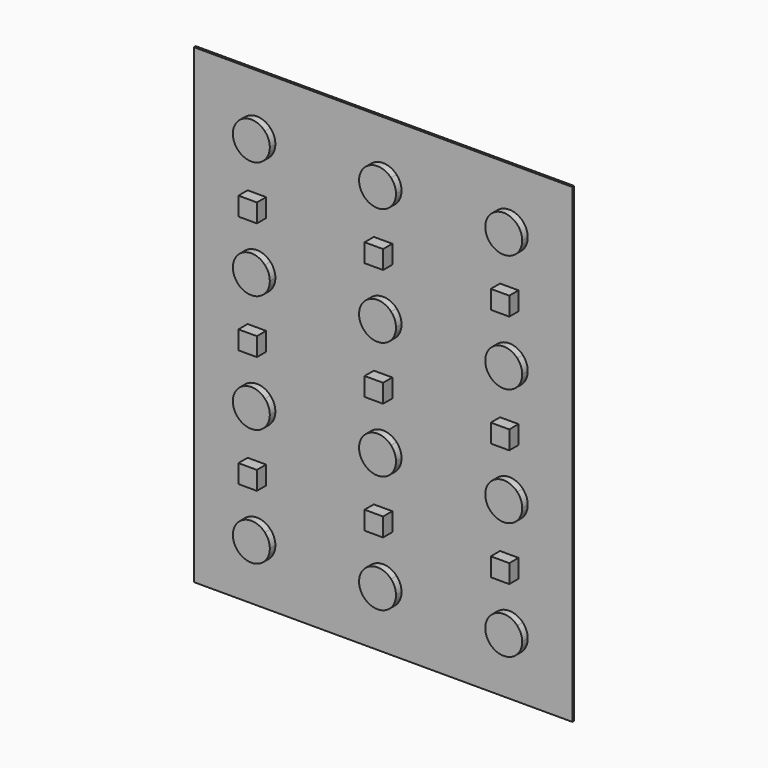
from build123d import *

# Parameters (mm, degrees)
F1_DEPTH = 3.175
F2_DEPTH = 12.7
F0_W     = 25.4
F0_H     = 12.7
F3_DEPTH = 19.05


# Not quite as in the source:
# - ends of sketch curves that miss each other by under 0.0002 mm in the source are joined


with BuildPart() as f1:
    # F0 (on Front) → F1 (new body)
    with BuildSketch(Plane.XZ):
        Polygon((-86.7833418, 323.85), (-260.35, 323.85), (-260.35, 161.925), (-186.2666709, 161.925), (-186.2666709, 174.625), (-160.8666709, 174.625), (-160.8666709, 161.925), (-86.7833418, 161.925), align=None)
        with BuildLine():
            ThreePointArc((-148.1666709, 242.8875), (-149.9350898056, 233.5757668112), (-154.9941020007, 225.5606513402))
            ThreePointArc((-154.9941020007, 225.5606513402), (-173.5666709, 217.4875), (-192.1392397993, 225.5606513402))
            ThreePointArc((-192.1392397993, 225.5606513402), (-198.9666709, 242.8875), (-192.1392397993, 260.2143486598))
            ThreePointArc((-192.1392397993, 260.2143486598), (-173.5666709, 268.2875), (-154.9941020007, 260.2143486598))
            ThreePointArc((-154.9941020007, 260.2143486598), (-149.9350898056, 252.1992331888), (-148.1666709, 242.8875))
        make_face(mode=Mode.SUBTRACT)
        Polygon((-186.2666709, 161.925), (-260.35, 161.925), (-260.35, 0), (-186.2666709, 0), (-186.2666709, 12.7), (-160.8666709, 12.7), (-160.8666709, 0), (-86.7833418, 0), (-86.7833418, 161.925), (-160.8666709, 161.925), (-160.8666709, 149.225), (-186.2666709, 149.225), align=None)
        with BuildLine():
            ThreePointArc((-154.9941020007, 63.6356513402), (-173.5666709, 55.5625), (-192.1392397993, 63.6356513402))
            ThreePointArc((-192.1392397993, 63.6356513402), (-198.9666709, 80.9625), (-192.1392397993, 98.2893486598))
            ThreePointArc((-192.1392397993, 98.2893486598), (-173.5666709, 106.3625), (-154.9941020007, 98.2893486598))
            ThreePointArc((-154.9941020007, 98.2893486598), (-149.9350898056, 90.2742331888), (-148.1666709, 80.9625))
            ThreePointArc((-148.1666709, 80.9625), (-149.9350898056, 71.6507668112), (-154.9941020007, 63.6356513402))
        make_face(mode=Mode.SUBTRACT)
        Polygon((-12.7, 161.925), (-86.7833418, 161.925), (-86.7833418, 0), (-12.7, 0), (-12.7, 12.7), (12.7, 12.7), (12.7, 0), (86.78332402, 0), (86.78332402, 161.925), (12.7, 161.925), (12.7, 149.225), (-12.7, 149.225), align=None)
        with BuildLine():
            ThreePointArc((18.5725583517, 63.6356536473), (-1.11224e-05, 55.5625), (-18.5725815993, 63.6356513402))
            ThreePointArc((-18.5725815993, 63.6356513402), (-25.4000127, 80.9625010214), (-18.5725802058, 98.2893501535))
            ThreePointArc((-18.5725802058, 98.2893501535), (-1.16786e-05, 106.3625), (18.5725561993, 98.2893486598))
            ThreePointArc((18.5725561993, 98.2893486598), (23.6315683944, 90.2742331888), (25.3999873, 80.9625))
            ThreePointArc((25.3999873, 80.9625), (23.6315689728, 71.650768279), (18.5725583517, 63.6356536473))
        make_face(mode=Mode.SUBTRACT)
        Polygon((86.78332402, 323.85), (-86.7833418, 323.85), (-86.7833418, 161.925), (-12.7, 161.925), (-12.7, 174.625), (12.7, 174.625), (12.7, 161.925), (86.78332402, 161.925), align=None)
        with BuildLine():
            ThreePointArc((25.399989205, 242.8874982228), (23.6315702994, 233.575765034), (18.5725581043, 225.560649563))
            ThreePointArc((18.5725581043, 225.560649563), (-1.10731e-05, 217.4874982228), (-18.5725800737, 225.5606499697))
            ThreePointArc((-18.5725800737, 225.5606499697), (-17.3268590481, 261.4600675015), (18.5725584837, 260.2143464759))
            ThreePointArc((18.5725584837, 260.2143464759), (23.6315704014, 252.1992311528), (25.399989205, 242.8874982228))
        make_face(mode=Mode.SUBTRACT)
        Polygon((260.35, 323.85), (86.78332402, 323.85), (86.78332402, 161.925), (160.86666201, 161.925), (160.86666201, 174.625), (186.26666201, 174.625), (186.26666201, 161.925), (260.35, 161.925), align=None)
        with BuildLine():
            ThreePointArc((198.96666201, 242.8875), (182.8783931272, 219.2559180893), (154.994090073, 225.5606545963))
            ThreePointArc((154.994090073, 225.5606545963), (148.16666201, 242.8875015776), (154.9940922253, 260.2143477108))
            ThreePointArc((154.9940922253, 260.2143477108), (173.5666609886, 268.2875), (192.1392304011, 260.2143492045))
            ThreePointArc((192.1392304011, 260.2143492045), (197.1982429678, 252.1992335353), (198.96666201, 242.8875))
        make_face(mode=Mode.SUBTRACT)
        Polygon((160.86666201, 0), (86.78332402, 0), (86.78332402, -161.925), (160.86666201, -161.925), (160.86666201, -149.225), (186.26666201, -149.225), (186.26666201, -161.925), (260.35, -161.925), (260.35, 0), (186.26666201, 0), (186.26666201, -12.7), (160.86666201, -12.7), align=None)
        with BuildLine():
            ThreePointArc((192.1392317947, -98.2893477108), (173.56666201, -106.3625), (154.9940922253, -98.2893477108))
            ThreePointArc((154.9940922253, -98.2893477108), (148.16666201, -80.9625), (154.9940922253, -63.6356522892))
            ThreePointArc((154.9940922253, -63.6356522892), (173.56666201, -55.5625), (192.1392317947, -63.6356522892))
            ThreePointArc((192.1392317947, -63.6356522892), (197.1982433423, -71.650767415), (198.96666201, -80.9625))
            ThreePointArc((198.96666201, -80.9625), (197.1982433423, -90.274232585), (192.1392317947, -98.2893477108))
        make_face(mode=Mode.SUBTRACT)
        Polygon((160.86666201, 161.925), (86.78332402, 161.925), (86.78332402, 0), (160.86666201, 0), (160.86666201, 12.7), (186.26666201, 12.7), (186.26666201, 0), (260.35, 0), (260.35, 161.925), (186.26666201, 161.925), (186.26666201, 149.225), (160.86666201, 149.225), align=None)
        with BuildLine():
            ThreePointArc((192.1392321741, 63.6356491414), (173.5666609886, 55.5624964455), (154.9940904524, 63.6356506351))
            ThreePointArc((154.9940904524, 63.6356506351), (148.16666201, 80.962497467), (154.9940918459, 98.2893437497))
            ThreePointArc((154.9940918459, 98.2893437497), (173.5666604324, 106.3624964455), (192.1392300217, 98.2893460568))
            ThreePointArc((192.1392300217, 98.2893460568), (197.1982428659, 90.2742302396), (198.96666201, 80.9624964455))
            ThreePointArc((198.96666201, 80.9624964455), (197.1982434443, 71.6507641193), (192.1392321741, 63.6356491414))
        make_face(mode=Mode.SUBTRACT)
        Polygon((-12.7, 0), (-86.7833418, 0), (-86.7833418, -161.925), (-12.7, -161.925), (-12.7, -149.225), (12.7, -149.225), (12.7, -161.925), (86.78332402, -161.925), (86.78332402, 0), (12.7, 0), (12.7, -12.7), (-12.7, -12.7), align=None)
        with BuildLine():
            ThreePointArc((18.5725603887, -98.2893482531), (-8.89e-06, -106.3625), (-18.5725781687, -98.2893482531))
            ThreePointArc((-18.5725781687, -98.2893482531), (-25.40000889, -80.9625), (-18.5725781687, -63.6356517469))
            ThreePointArc((-18.5725781687, -63.6356517469), (-8.89e-06, -55.5625), (18.5725603887, -63.6356517469))
            ThreePointArc((18.5725603887, -63.6356517469), (23.6315723064, -71.65076707), (25.39999111, -80.9625))
            ThreePointArc((25.39999111, -80.9625), (23.6315723064, -90.27423293), (18.5725603887, -98.2893482531))
        make_face(mode=Mode.SUBTRACT)
        Polygon((-186.2666709, 0), (-260.35, 0), (-260.35, -161.925), (-186.2666709, -161.925), (-186.2666709, -149.225), (-160.8666709, -149.225), (-160.8666709, -161.925), (-86.7833418, -161.925), (-86.7833418, 0), (-160.8666709, 0), (-160.8666709, -12.7), (-186.2666709, -12.7), align=None)
        with BuildLine():
            ThreePointArc((-154.9941020007, -98.2893486598), (-173.5666709, -106.3625), (-192.1392397993, -98.2893486598))
            ThreePointArc((-192.1392397993, -98.2893486598), (-198.9666709, -80.9625), (-192.1392397993, -63.6356513402))
            ThreePointArc((-192.1392397993, -63.6356513402), (-173.5666709, -55.5625), (-154.9941020007, -63.6356513402))
            ThreePointArc((-154.9941020007, -63.6356513402), (-149.9350898056, -71.6507668112), (-148.1666709, -80.9625))
            ThreePointArc((-148.1666709, -80.9625), (-149.9350898056, -90.2742331888), (-154.9941020007, -98.2893486598))
        make_face(mode=Mode.SUBTRACT)
        Polygon((-186.2666709, -161.925), (-260.35, -161.925), (-260.35, -323.85), (-86.7833418, -323.85), (-86.7833418, -161.925), (-160.8666709, -161.925), (-160.8666709, -174.625), (-186.2666709, -174.625), align=None)
        with BuildLine():
            ThreePointArc((-154.9941020007, -260.2143486598), (-173.5666709, -268.2875), (-192.1392397993, -260.2143486598))
            ThreePointArc((-192.1392397993, -260.2143486598), (-198.9666709, -242.8875), (-192.1392397993, -225.5606513402))
            ThreePointArc((-192.1392397993, -225.5606513402), (-173.5666709, -217.4875), (-154.9941020007, -225.5606513402))
            ThreePointArc((-154.9941020007, -225.5606513402), (-149.9350898056, -233.5757668112), (-148.1666709, -242.8875))
            ThreePointArc((-148.1666709, -242.8875), (-149.9350898056, -252.1992331888), (-154.9941020007, -260.2143486598))
        make_face(mode=Mode.SUBTRACT)
        Polygon((-12.7, -161.925), (-86.7833418, -161.925), (-86.7833418, -323.85), (86.78332402, -323.85), (86.78332402, -161.925), (12.7, -161.925), (12.7, -174.625), (-12.7, -174.625), align=None)
        with BuildLine():
            ThreePointArc((-18.5725781687, -260.2143482531), (-25.40000889, -242.8875), (-18.5725781687, -225.5606517469))
            ThreePointArc((-18.5725781687, -225.5606517469), (-8.89e-06, -217.4875), (18.5725603887, -225.5606517469))
            ThreePointArc((18.5725603887, -225.5606517469), (23.6315723064, -233.57576707), (25.39999111, -242.8875))
            ThreePointArc((25.39999111, -242.8875), (23.6315723064, -252.19923293), (18.5725603887, -260.2143482531))
            ThreePointArc((18.5725603887, -260.2143482531), (-8.89e-06, -268.2875), (-18.5725781687, -260.2143482531))
        make_face(mode=Mode.SUBTRACT)
        Polygon((160.86666201, -161.925), (86.78332402, -161.925), (86.78332402, -323.85), (260.35, -323.85), (260.35, -161.925), (186.26666201, -161.925), (186.26666201, -174.625), (160.86666201, -174.625), align=None)
        with BuildLine():
            ThreePointArc((154.9940922253, -225.5606522892), (173.56666201, -217.4875), (192.1392317947, -225.5606522892))
            ThreePointArc((192.1392317947, -225.5606522892), (197.1982433423, -233.575767415), (198.96666201, -242.8875))
            ThreePointArc((198.96666201, -242.8875), (197.1982433423, -252.199232585), (192.1392317947, -260.2143477108))
            ThreePointArc((192.1392317947, -260.2143477108), (173.56666201, -268.2875), (154.9940922253, -260.2143477108))
            ThreePointArc((154.9940922253, -260.2143477108), (148.16666201, -242.8875), (154.9940922253, -225.5606522892))
        make_face(mode=Mode.SUBTRACT)
    extrude(amount=F1_DEPTH)

    # F0 (on Front) → F2 (join)
    with BuildSketch(Plane.XZ):
        with BuildLine():
            Line((-192.1392397993, 260.2143486598), (-173.5666709, 242.8875))
            Line((-173.5666709, 242.8875), (-154.9941020007, 260.2143486598))
            ThreePointArc((-154.9941020007, 260.2143486598), (-173.5666709, 268.2875), (-192.1392397993, 260.2143486598))
        make_face()
        with BuildLine():
            Line((-192.1392397993, 225.5606513402), (-173.5666709, 242.8875))
            Line((-173.5666709, 242.8875), (-192.1392397993, 260.2143486598))
            ThreePointArc((-192.1392397993, 260.2143486598), (-198.9666709, 242.8875), (-192.1392397993, 225.5606513402))
        make_face()
        with BuildLine():
            ThreePointArc((-192.1392397993, 225.5606513402), (-173.5666709, 217.4875), (-154.9941020007, 225.5606513402))
            Line((-154.9941020007, 225.5606513402), (-173.5666709, 242.8875))
            Line((-173.5666709, 242.8875), (-192.1392397993, 225.5606513402))
        make_face()
        with BuildLine():
            Line((-173.5666709, 242.8875), (-154.9941020007, 225.5606513402))
            ThreePointArc((-154.9941020007, 225.5606513402), (-149.9350898056, 233.5757668112), (-148.1666709, 242.8875))
            ThreePointArc((-148.1666709, 242.8875), (-149.9350898056, 252.1992331888), (-154.9941020007, 260.2143486598))
            Line((-154.9941020007, 260.2143486598), (-173.5666709, 242.8875))
        make_face()
        with BuildLine():
            Line((-18.5725800737, 225.5606499697), (-1.0795e-05, 242.8874982228))
            Line((-1.0795e-05, 242.8874982228), (18.5725584837, 260.2143464759))
            ThreePointArc((18.5725584837, 260.2143464759), (-17.3268590481, 261.4600675015), (-18.5725800737, 225.5606499697))
        make_face()
        with BuildLine():
            Line((18.5725584837, 260.2143464759), (-1.0795e-05, 242.8874982228))
            Line((-1.0795e-05, 242.8874982228), (18.5725581043, 225.560649563))
            ThreePointArc((18.5725581043, 225.560649563), (23.6315702994, 233.575765034), (25.399989205, 242.8874982228))
            ThreePointArc((25.399989205, 242.8874982228), (23.6315704014, 252.1992311528), (18.5725584837, 260.2143464759))
        make_face()
        with BuildLine():
            Line((18.5725581043, 225.560649563), (-1.0795e-05, 242.8874982228))
            Line((-1.0795e-05, 242.8874982228), (-18.5725800737, 225.5606499697))
            ThreePointArc((-18.5725800737, 225.5606499697), (-1.10731e-05, 217.4874982228), (18.5725581043, 225.560649563))
        make_face()
        with BuildLine():
            Line((154.9940922253, 260.2143477108), (173.56666201, 242.8875))
            Line((173.56666201, 242.8875), (192.1392304011, 260.2143492045))
            ThreePointArc((192.1392304011, 260.2143492045), (173.5666609886, 268.2875), (154.9940922253, 260.2143477108))
        make_face()
        with BuildLine():
            ThreePointArc((154.9940922253, 260.2143477108), (148.16666201, 242.8875015776), (154.994090073, 225.5606545963))
            Line((154.994090073, 225.5606545963), (173.566660237, 242.8875019004))
            Line((173.566660237, 242.8875019004), (154.9940922253, 260.2143477108))
        make_face()
        with BuildLine():
            Line((173.566660237, 242.8875019004), (154.994090073, 225.5606545963))
            ThreePointArc((154.994090073, 225.5606545963), (182.8783931272, 219.2559180893), (198.96666201, 242.8875))
            ThreePointArc((198.96666201, 242.8875), (197.1982429678, 252.1992335353), (192.1392304011, 260.2143492045))
            Line((192.1392304011, 260.2143492045), (173.566660237, 242.8875019004))
        make_face()
        with BuildLine():
            Line((154.9940918459, 98.2893437497), (173.566660105, 80.9624982228))
            Line((173.566660105, 80.9624982228), (192.1392300217, 98.2893460568))
            ThreePointArc((192.1392300217, 98.2893460568), (173.5666604324, 106.3624964455), (154.9940918459, 98.2893437497))
        make_face()
        with BuildLine():
            ThreePointArc((154.9940918459, 98.2893437497), (148.16666201, 80.962497467), (154.9940904524, 63.6356506351))
            Line((154.9940904524, 63.6356506351), (173.566660105, 80.9624982228))
            Line((173.566660105, 80.9624982228), (154.9940918459, 98.2893437497))
        make_face()
        with BuildLine():
            Line((173.566660105, 80.9624982228), (154.9940904524, 63.6356506351))
            ThreePointArc((154.9940904524, 63.6356506351), (173.5666609886, 55.5624964455), (192.1392321741, 63.6356491414))
            Line((192.1392321741, 63.6356491414), (173.566660105, 80.9624982228))
        make_face()
        with BuildLine():
            Line((192.1392300217, 98.2893460568), (173.566660105, 80.9624982228))
            Line((173.566660105, 80.9624982228), (192.1392321741, 63.6356491414))
            ThreePointArc((192.1392321741, 63.6356491414), (197.1982434443, 71.6507641193), (198.96666201, 80.9624964455))
            ThreePointArc((198.96666201, 80.9624964455), (197.1982428659, 90.2742302396), (192.1392300217, 98.2893460568))
        make_face()
        with BuildLine():
            Line((18.5725561993, 98.2893486598), (-1.0795e-05, 80.9625017772))
            Line((-1.0795e-05, 80.9625017772), (18.5725583517, 63.6356536473))
            ThreePointArc((18.5725583517, 63.6356536473), (23.6315689728, 71.650768279), (25.3999873, 80.9625))
            ThreePointArc((25.3999873, 80.9625), (23.6315683944, 90.2742331888), (18.5725561993, 98.2893486598))
        make_face()
        with BuildLine():
            Line((-18.5725802058, 98.2893501535), (-1.0795e-05, 80.9625017772))
            Line((-1.0795e-05, 80.9625017772), (18.5725561993, 98.2893486598))
            ThreePointArc((18.5725561993, 98.2893486598), (-1.16786e-05, 106.3625), (-18.5725802058, 98.2893501535))
        make_face()
        with BuildLine():
            ThreePointArc((-18.5725802058, 98.2893501535), (-25.4000127, 80.9625010214), (-18.5725815993, 63.6356513402))
            Line((-18.5725815993, 63.6356513402), (-1.0795e-05, 80.9625017772))
            Line((-1.0795e-05, 80.9625017772), (-18.5725802058, 98.2893501535))
        make_face()
        with BuildLine():
            Line((-1.0795e-05, 80.9625017772), (-18.5725815993, 63.6356513402))
            ThreePointArc((-18.5725815993, 63.6356513402), (-1.11224e-05, 55.5625), (18.5725583517, 63.6356536473))
            Line((18.5725583517, 63.6356536473), (-1.0795e-05, 80.9625017772))
        make_face()
        with BuildLine():
            Line((-173.5666709, 80.9625), (-192.1392397993, 63.6356513402))
            ThreePointArc((-192.1392397993, 63.6356513402), (-173.5666709, 55.5625), (-154.9941020007, 63.6356513402))
            Line((-154.9941020007, 63.6356513402), (-173.5666709, 80.9625))
        make_face()
        with BuildLine():
            Line((-154.9941020007, 98.2893486598), (-173.5666709, 80.9625))
            Line((-173.5666709, 80.9625), (-154.9941020007, 63.6356513402))
            ThreePointArc((-154.9941020007, 63.6356513402), (-149.9350898056, 71.6507668112), (-148.1666709, 80.9625))
            ThreePointArc((-148.1666709, 80.9625), (-149.9350898056, 90.2742331888), (-154.9941020007, 98.2893486598))
        make_face()
        with BuildLine():
            Line((-192.1392397993, 98.2893486598), (-173.5666709, 80.9625))
            Line((-173.5666709, 80.9625), (-154.9941020007, 98.2893486598))
            ThreePointArc((-154.9941020007, 98.2893486598), (-173.5666709, 106.3625), (-192.1392397993, 98.2893486598))
        make_face()
        with BuildLine():
            ThreePointArc((-192.1392397993, 98.2893486598), (-198.9666709, 80.9625), (-192.1392397993, 63.6356513402))
            Line((-192.1392397993, 63.6356513402), (-173.5666709, 80.9625))
            Line((-173.5666709, 80.9625), (-192.1392397993, 98.2893486598))
        make_face()
        with BuildLine():
            Line((-192.1392397993, -63.6356513402), (-173.5666709, -80.9625))
            Line((-173.5666709, -80.9625), (-154.9941020007, -63.6356513402))
            ThreePointArc((-154.9941020007, -63.6356513402), (-173.5666709, -55.5625), (-192.1392397993, -63.6356513402))
        make_face()
        with BuildLine():
            Line((-154.9941020007, -63.6356513402), (-173.5666709, -80.9625))
            Line((-173.5666709, -80.9625), (-154.9941020007, -98.2893486598))
            ThreePointArc((-154.9941020007, -98.2893486598), (-149.9350898056, -90.2742331888), (-148.1666709, -80.9625))
            ThreePointArc((-148.1666709, -80.9625), (-149.9350898056, -71.6507668112), (-154.9941020007, -63.6356513402))
        make_face()
        with BuildLine():
            Line((-173.5666709, -80.9625), (-192.1392397993, -98.2893486598))
            ThreePointArc((-192.1392397993, -98.2893486598), (-173.5666709, -106.3625), (-154.9941020007, -98.2893486598))
            Line((-154.9941020007, -98.2893486598), (-173.5666709, -80.9625))
        make_face()
        with BuildLine():
            ThreePointArc((-192.1392397993, -63.6356513402), (-198.9666709, -80.9625), (-192.1392397993, -98.2893486598))
            Line((-192.1392397993, -98.2893486598), (-173.5666709, -80.9625))
            Line((-173.5666709, -80.9625), (-192.1392397993, -63.6356513402))
        make_face()
        with BuildLine():
            Line((-18.5725781687, -63.6356517469), (-8.89e-06, -80.9625))
            Line((-8.89e-06, -80.9625), (18.5725603887, -63.6356517469))
            ThreePointArc((18.5725603887, -63.6356517469), (-8.89e-06, -55.5625), (-18.5725781687, -63.6356517469))
        make_face()
        with BuildLine():
            ThreePointArc((-18.5725781687, -63.6356517469), (-25.40000889, -80.9625), (-18.5725781687, -98.2893482531))
            Line((-18.5725781687, -98.2893482531), (-8.89e-06, -80.9625))
            Line((-8.89e-06, -80.9625), (-18.5725781687, -63.6356517469))
        make_face()
        with BuildLine():
            Line((-8.89e-06, -80.9625), (-18.5725781687, -98.2893482531))
            ThreePointArc((-18.5725781687, -98.2893482531), (-8.89e-06, -106.3625), (18.5725603887, -98.2893482531))
            Line((18.5725603887, -98.2893482531), (-8.89e-06, -80.9625))
        make_face()
        with BuildLine():
            Line((18.5725603887, -63.6356517469), (-8.89e-06, -80.9625))
            Line((-8.89e-06, -80.9625), (18.5725603887, -98.2893482531))
            ThreePointArc((18.5725603887, -98.2893482531), (23.6315723064, -90.27423293), (25.39999111, -80.9625))
            ThreePointArc((25.39999111, -80.9625), (23.6315723064, -71.65076707), (18.5725603887, -63.6356517469))
        make_face()
        with BuildLine():
            Line((154.9940922253, -63.6356522892), (173.56666201, -80.9625))
            Line((173.56666201, -80.9625), (192.1392317947, -63.6356522892))
            ThreePointArc((192.1392317947, -63.6356522892), (173.56666201, -55.5625), (154.9940922253, -63.6356522892))
        make_face()
        with BuildLine():
            ThreePointArc((154.9940922253, -63.6356522892), (148.16666201, -80.9625), (154.9940922253, -98.2893477108))
            Line((154.9940922253, -98.2893477108), (173.56666201, -80.9625))
            Line((173.56666201, -80.9625), (154.9940922253, -63.6356522892))
        make_face()
        with BuildLine():
            Line((173.56666201, -80.9625), (154.9940922253, -98.2893477108))
            ThreePointArc((154.9940922253, -98.2893477108), (173.56666201, -106.3625), (192.1392317947, -98.2893477108))
            Line((192.1392317947, -98.2893477108), (173.56666201, -80.9625))
        make_face()
        with BuildLine():
            Line((192.1392317947, -63.6356522892), (173.56666201, -80.9625))
            Line((173.56666201, -80.9625), (192.1392317947, -98.2893477108))
            ThreePointArc((192.1392317947, -98.2893477108), (197.1982433423, -90.274232585), (198.96666201, -80.9625))
            ThreePointArc((198.96666201, -80.9625), (197.1982433423, -71.650767415), (192.1392317947, -63.6356522892))
        make_face()
        with BuildLine():
            Line((173.56666201, -242.8875), (192.1392317947, -225.5606522892))
            ThreePointArc((192.1392317947, -225.5606522892), (173.56666201, -217.4875), (154.9940922253, -225.5606522892))
            Line((154.9940922253, -225.5606522892), (173.56666201, -242.8875))
        make_face()
        with BuildLine():
            Line((154.9940922253, -260.2143477108), (173.56666201, -242.8875))
            Line((173.56666201, -242.8875), (154.9940922253, -225.5606522892))
            ThreePointArc((154.9940922253, -225.5606522892), (148.16666201, -242.8875), (154.9940922253, -260.2143477108))
        make_face()
        with BuildLine():
            Line((192.1392317947, -260.2143477108), (173.56666201, -242.8875))
            Line((173.56666201, -242.8875), (154.9940922253, -260.2143477108))
            ThreePointArc((154.9940922253, -260.2143477108), (173.56666201, -268.2875), (192.1392317947, -260.2143477108))
        make_face()
        with BuildLine():
            ThreePointArc((198.96666201, -242.8875), (197.1982433423, -233.575767415), (192.1392317947, -225.5606522892))
            Line((192.1392317947, -225.5606522892), (173.56666201, -242.8875))
            Line((173.56666201, -242.8875), (192.1392317947, -260.2143477108))
            ThreePointArc((192.1392317947, -260.2143477108), (197.1982433423, -252.199232585), (198.96666201, -242.8875))
        make_face()
        with BuildLine():
            Line((18.5725603887, -225.5606517469), (-8.89e-06, -242.8875))
            Line((-8.89e-06, -242.8875), (18.5725603887, -260.2143482531))
            ThreePointArc((18.5725603887, -260.2143482531), (23.6315723064, -252.19923293), (25.39999111, -242.8875))
            ThreePointArc((25.39999111, -242.8875), (23.6315723064, -233.57576707), (18.5725603887, -225.5606517469))
        make_face()
        with BuildLine():
            Line((18.5725603887, -260.2143482531), (-8.89e-06, -242.8875))
            Line((-8.89e-06, -242.8875), (-18.5725781687, -260.2143482531))
            ThreePointArc((-18.5725781687, -260.2143482531), (-8.89e-06, -268.2875), (18.5725603887, -260.2143482531))
        make_face()
        with BuildLine():
            ThreePointArc((18.5725603887, -225.5606517469), (-8.89e-06, -217.4875), (-18.5725781687, -225.5606517469))
            Line((-18.5725781687, -225.5606517469), (-8.89e-06, -242.8875))
            Line((-8.89e-06, -242.8875), (18.5725603887, -225.5606517469))
        make_face()
        with BuildLine():
            Line((-8.89e-06, -242.8875), (-18.5725781687, -225.5606517469))
            ThreePointArc((-18.5725781687, -225.5606517469), (-25.40000889, -242.8875), (-18.5725781687, -260.2143482531))
            Line((-18.5725781687, -260.2143482531), (-8.89e-06, -242.8875))
        make_face()
        with BuildLine():
            Line((-154.9941020007, -225.5606513402), (-173.5666709, -242.8875))
            Line((-173.5666709, -242.8875), (-154.9941020007, -260.2143486598))
            ThreePointArc((-154.9941020007, -260.2143486598), (-149.9350898056, -252.1992331888), (-148.1666709, -242.8875))
            ThreePointArc((-148.1666709, -242.8875), (-149.9350898056, -233.5757668112), (-154.9941020007, -225.5606513402))
        make_face()
        with BuildLine():
            Line((-173.5666709, -242.8875), (-192.1392397993, -260.2143486598))
            ThreePointArc((-192.1392397993, -260.2143486598), (-173.5666709, -268.2875), (-154.9941020007, -260.2143486598))
            Line((-154.9941020007, -260.2143486598), (-173.5666709, -242.8875))
        make_face()
        with BuildLine():
            ThreePointArc((-192.1392397993, -225.5606513402), (-198.9666709, -242.8875), (-192.1392397993, -260.2143486598))
            Line((-192.1392397993, -260.2143486598), (-173.5666709, -242.8875))
            Line((-173.5666709, -242.8875), (-192.1392397993, -225.5606513402))
        make_face()
        with BuildLine():
            Line((-192.1392397993, -225.5606513402), (-173.5666709, -242.8875))
            Line((-173.5666709, -242.8875), (-154.9941020007, -225.5606513402))
            ThreePointArc((-154.9941020007, -225.5606513402), (-173.5666709, -217.4875), (-192.1392397993, -225.5606513402))
        make_face()
    extrude(amount=F2_DEPTH)

    # F0 (on Front) → F3 (join)
    with BuildSketch(Plane.XZ):
        with Locations((-173.5666709, 168.275)):
            Rectangle(F0_W, F0_H)
        with Locations((-173.5666709, 155.575)):
            Rectangle(F0_W, F0_H)
        with Locations((0, 168.275)):
            Rectangle(F0_W, F0_H)
        with Locations((0, 155.575)):
            Rectangle(F0_W, F0_H)
        with Locations((173.56666201, 168.275)):
            Rectangle(F0_W, F0_H)
        with Locations((173.56666201, 155.575)):
            Rectangle(F0_W, F0_H)
        with Locations((173.56666201, 6.35)):
            Rectangle(F0_W, F0_H)
        with Locations((173.56666201, -6.35)):
            Rectangle(F0_W, F0_H)
        with Locations((0, 6.35)):
            Rectangle(F0_W, F0_H)
        with Locations((0, -6.35)):
            Rectangle(F0_W, F0_H)
        with Locations((-173.5666709, 6.35)):
            Rectangle(F0_W, F0_H)
        with Locations((-173.5666709, -6.35)):
            Rectangle(F0_W, F0_H)
        with Locations((-173.5666709, -155.575)):
            Rectangle(F0_W, F0_H)
        with Locations((-173.5666709, -168.275)):
            Rectangle(F0_W, F0_H)
        with Locations((0, -155.575)):
            Rectangle(F0_W, F0_H)
        with Locations((0, -168.275)):
            Rectangle(F0_W, F0_H)
        with Locations((173.56666201, -155.575)):
            Rectangle(F0_W, F0_H)
        with Locations((173.56666201, -168.275)):
            Rectangle(F0_W, F0_H)
    extrude(amount=F3_DEPTH)


solid = f1.part
